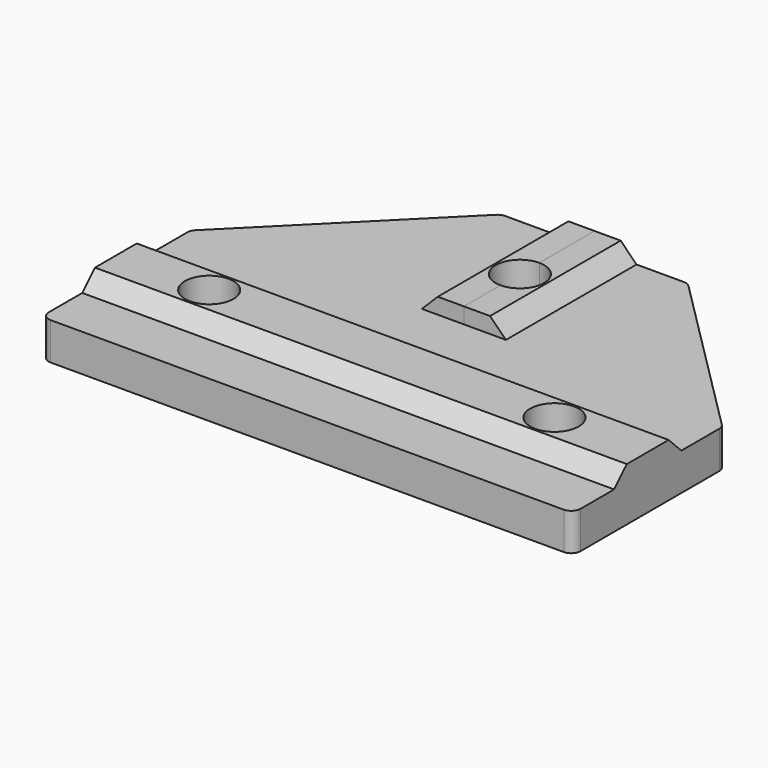
from build123d import *

# Parameters (mm, degrees)
F0_R     = 2.6
F1_DEPTH = 4
F2_W     = 28.5
F2_H     = 9
F2_R     = 2.6
F3_DEPTH = 1.7
F4_SIZE  = 1.69999
F5_R     = 1


# Not quite as in the source:
# - a fillet or chamfer is up to 0.001 mm smaller than in the source, because OpenCascade refuses the exact size


with BuildPart() as f1:
    # F0 (on Top) → F1 (new body)
    with BuildSketch(Plane.XY):
        with BuildLine():
            Line((-28.5, 0), (0, 0))
            Line((0, 0), (0, 25.9))
            ThreePointArc((0, 25.9), (-2.6, 28.5), (0, 31.1))
            Line((0, 31.1), (0, 38.5))
            Line((0, 38.5), (-10, 38.5))
            Line((-10, 38.5), (-28.5, 20))
            Line((-28.5, 20), (-28.5, 0))
        make_face()
        with Locations((-18.5, 10)):
            Circle(F0_R, mode=Mode.SUBTRACT)
    extrude(amount=F1_DEPTH)

    # F2 (on face) → F3 (join)
    with BuildSketch(Plane.XY.offset(4)):
        with Locations((-14.25, 10)):
            Rectangle(F2_W, F2_H)
        with Locations((-18.5, 10)):
            Circle(F2_R, mode=Mode.SUBTRACT)
        with BuildLine():
            ThreePointArc((0, 25.9), (-2.6, 28.5), (0, 31.1))
            Line((0, 31.1), (0, 38.5))
            Line((0, 38.5), (-4.5, 38.5))
            Line((-4.5, 38.5), (-4.5, 21))
            Line((-4.5, 21), (0, 21))
            Line((0, 21), (0, 25.9))
        make_face()
    extrude(amount=F3_DEPTH)

    # F4 (size 1.7 in the source; OpenCascade refuses exactly that, so slightly less here)
    f4_edges = [f1.edges().sort_by_distance(p)[0] for p in [
        (-14.25, 14.5, 5.7),
        (-14.25, 5.5, 5.7),
        (-4.5, 29.75, 5.7),
    ]]
    chamfer(f4_edges, length=F4_SIZE)

    # F5
    f5_edges = [f1.edges().sort_by_distance(p)[0] for p in [
        (-10, 38.5, 2),
        (-28.5, 20, 2),
        (-28.5, 0, 2),
    ]]
    fillet(f5_edges, radius=F5_R)

    # F6: F1 across face


with BuildPart() as f1_1:
    add(f1.part)
    add(f1.part.mirror(Plane(origin=(0, 34.8, 2.85), x_dir=(0, 1, 0), z_dir=(1, 0, 0))))


solid = f1_1.part
